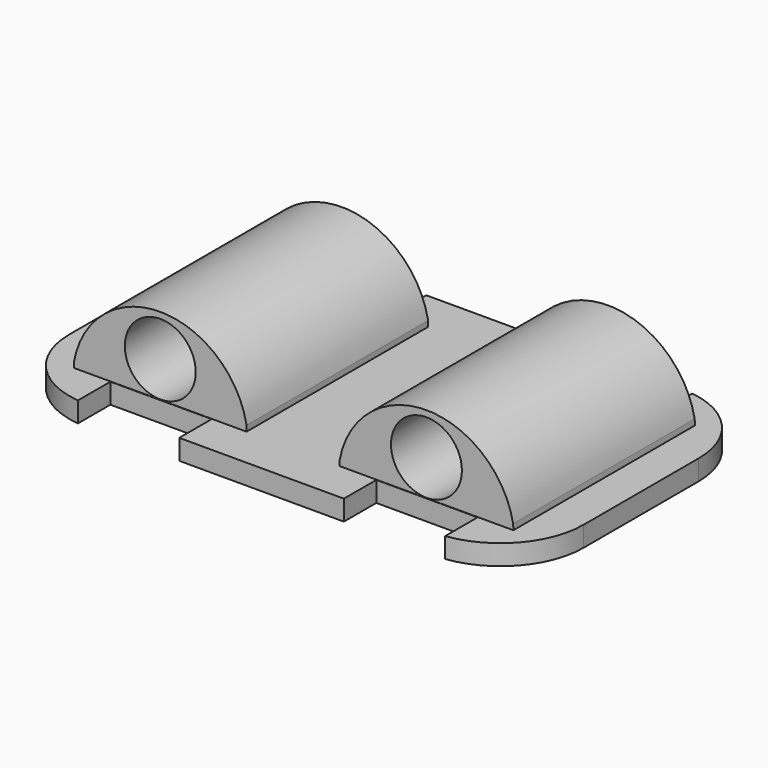
from build123d import *

# Parameters (mm, degrees)
F1_DEPTH    = 0.5
F2_R        = 1.75
F3_DEPTH    = 5.6
F4_T1_DEPTH = 21.3501190522
F4_T3_DEPTH = 21.4204938405


# Not quite as in the source:
# - a fillet or chamfer that OpenCascade refuses, or shapes differently, is made with other operations: its cross-section is extruded or revolved along the edge and cut away or added


with BuildPart() as f1:
    # F0 (on Top) → F1 (new body, symmetric)
    with BuildSketch(Plane.XY):
        Polygon((12.7, -7.62), (12.7, 7.62), (9.1240987852, 7.62), (9.1240987852, 5.62), (4.1240987852, 5.62), (4.1240987852, 7.62), (-4.0011659991, 7.62), (-4.0011659991, 5.62), (-9.0011659991, 5.62), (-9.0011659991, 7.62), (-12.7, 7.62), (-12.7, -7.62), (-9.0011659991, -7.62), (-9.0011659991, -5.62), (-4.0011659991, -5.62), (-4.0011659991, -7.62), (4.1240987852, -7.62), (4.1240987852, -5.62), (9.1240987852, -5.62), (9.1240987852, -7.62), align=None)
    extrude(amount=F1_DEPTH, both=True)

    # F2 (on Front) → F3 (join, symmetric)
    with BuildSketch(Plane.XZ):
        with BuildLine():
            Line((-2.2954130392, -0.004001643), (-2.2954130392, 0.7802180896))
            ThreePointArc((-2.2954130392, 0.7802180896), (-6.588071973, 4.326288954), (-10.8247913043, 0.7135685656))
            Line((-10.8247913043, 0.7135685656), (-10.8191841297, -0.004001643))
            Line((-10.8191841297, -0.004001643), (-6.5542345937, -0.004001643))
            Line((-6.5542345937, -0.004001643), (-2.2954130392, -0.004001643))
        make_face()
        with Locations((-6.5542345937, 2.2683413699)):
            Circle(F2_R, mode=Mode.SUBTRACT)
        with BuildLine():
            Line((10.8930142596, 0), (10.861883565, 0.7857921351))
            ThreePointArc((10.861883565, 0.7857921351), (6.5823484291, 4.3273176658), (2.3028132932, 0.7857921351))
            Line((2.3028132932, 0.7857921351), (2.3028132932, 0))
            Line((2.3028132932, 0), (10.8930142596, 0))
        make_face()
        with Locations((6.5823484291, 2.2683413699)):
            Circle(F2_R, mode=Mode.SUBTRACT)
    extrude(amount=F3_DEPTH, both=True)

    # F4: fillet of radius 4.104163056 on 4 edges, made by hand

    # F4_s2 → F4_t1 (cut)
    with BuildSketch(Plane.XY.offset(-10.6750595261)):
        with BuildLine():
            ThreePointArc((9.1240987852, -7.62), (11.6790355366, -6.2588580306), (12.7, -3.5499761896))
            Line((12.7, -3.5499761896), (12.7, -7.62))
            Line((12.7, -7.62), (9.1240987852, -7.62))
        make_face()
        with BuildLine():
            ThreePointArc((12.7, 3.5499761896), (11.6790355366, 6.2588580306), (9.1240987852, 7.62))
            Line((9.1240987852, 7.62), (12.7, 7.62))
            Line((12.7, 7.62), (12.7, 3.5499761896))
        make_face()
    extrude(amount=F4_T1_DEPTH, mode=Mode.SUBTRACT)

    # F4_s4 → F4_t3 (cut)
    with BuildSketch(Plane.XY.offset(-10.7102469202)):
        with BuildLine():
            ThreePointArc((-9.0011659991, 7.62), (-11.6378503335, 6.2909527611), (-12.7, 3.5359012319))
            Line((-12.7, 3.5359012319), (-12.7, 7.62))
            Line((-12.7, 7.62), (-9.0011659991, 7.62))
        make_face()
        with BuildLine():
            ThreePointArc((-12.7, -3.5359012319), (-11.6378503335, -6.2909527611), (-9.0011659991, -7.62))
            Line((-9.0011659991, -7.62), (-12.7, -7.62))
            Line((-12.7, -7.62), (-12.7, -3.5359012319))
        make_face()
    extrude(amount=F4_T3_DEPTH, mode=Mode.SUBTRACT)


solid = f1.part
